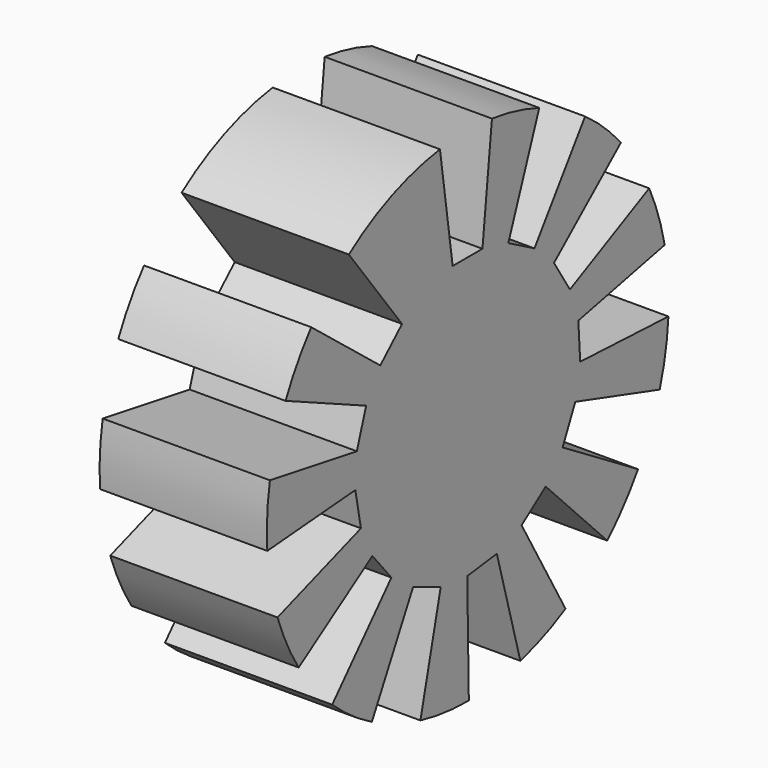
from build123d import *

# Parameters (mm, degrees)
F0_W            = 28.2793976367
F0_H            = 42.4683615565
F3_DEPTH        = 50.8
F3_COPIES_COUNT = 12
F3_COPIES_ANGLE = 316.8


# Not quite as in the source:
# - a feature of the source that left no trace in its solid (it failed there, or was rolled back) is left out
# - a pattern or mirror of a feature is missing from the dataset's text; its kind, count and spacing are read off the source's solid


with BuildPart() as f1:
    # F0 (on Front) → F1 (revolve)
    with BuildSketch(Plane.XZ):
        with Locations((-14.1396988183, 21.2341807783)):
            Rectangle(F0_W, F0_H)
    revolve(axis=Axis((-14.1396988183, 0, 0), (-1, 0, 0)))

    # F2 (on face) → F3 (cut)
    with BuildSketch(Plane(origin=(-28.2793976367, 0, 0), x_dir=(0, -1, 0), z_dir=(-1, 0, 0))):
        with BuildLine():
            ThreePointArc((5.8825213519, 42.0589785401), (0.3916223416, 42.4665558438), (-5.1058594535, 42.1603122917))
            Line((-5.1058594535, 42.1603122917), (-3.0962699093, 23.6033536494))
            Line((-3.0962699093, 23.6033536494), (0, 23.6033536494))
            Line((0, 23.6033536494), (3.2008844428, 23.6033536494))
            Line((3.2008844428, 23.6033536494), (5.8825213519, 42.0589785401))
        make_face()
    f3 = extrude(amount=-F3_DEPTH, mode=Mode.SUBTRACT)

    # F3_copies: F3 ×12 about axis
    f3_copies_axis = Axis((0, 0, 0), (-1, 0, 0))
    for i in range(1, F3_COPIES_COUNT):
        add(f3.rotate(f3_copies_axis, i * F3_COPIES_ANGLE / (F3_COPIES_COUNT - 1)), mode=Mode.SUBTRACT)


solid = f1.part
